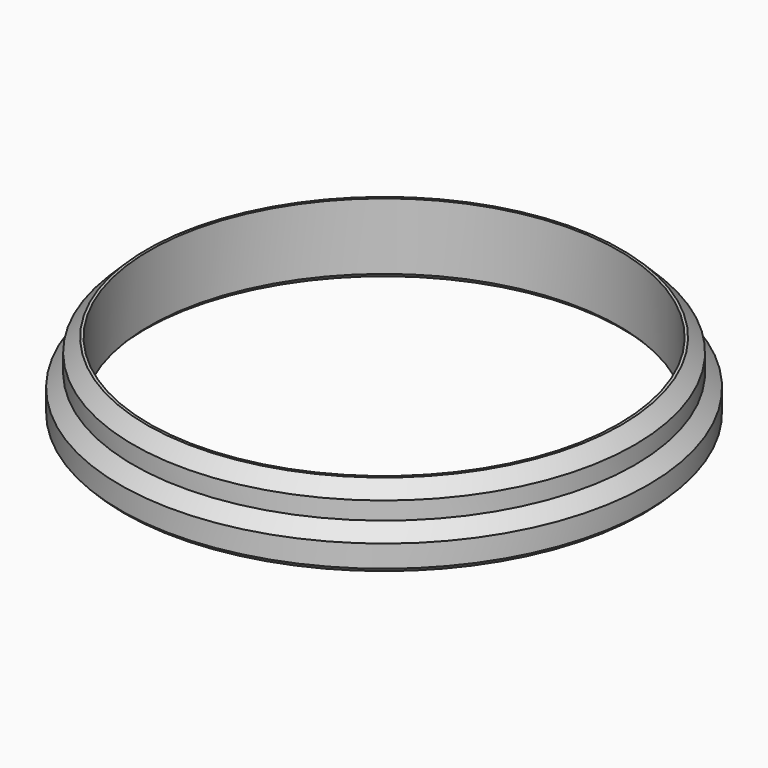
from build123d import *

# Parameters (mm, degrees)
F0_R     = 28.3
F0_R_2   = 26.5
F1_DEPTH = 8
F2_SIZE  = 1.5
F3_SIZE  = 0.5
F4_R     = 29.8
F4_R_2   = 28.3
F5_DEPTH = 4.5
F6_SIZE  = 1.49999
F7_SIZE  = 0.5


# Not quite as in the source:
# - a fillet or chamfer is up to 0.001 mm smaller than in the source, because OpenCascade refuses the exact size


with BuildPart() as f1:
    # F0 (on Top) → F1 (new body)
    with BuildSketch(Plane.XY):
        Circle(F0_R)
        Circle(F0_R_2, mode=Mode.SUBTRACT)
    extrude(amount=F1_DEPTH)

    # F2
    f2_edges = [f1.edges().sort_by_distance(p)[0] for p in [
        (-28.3, 0, 8),
    ]]
    chamfer(f2_edges, length=F2_SIZE)

    # F3
    f3_edges = [f1.edges().sort_by_distance(p)[0] for p in [
        (-26.5, 0, 0),
    ]]
    chamfer(f3_edges, length=F3_SIZE)

    # F4 (on face) → F5 (join)
    with BuildSketch(Plane(origin=(0, 0, 0), x_dir=(1, 0, 0), z_dir=(0, 0, -1))):
        Circle(F4_R)
        Circle(F4_R_2, mode=Mode.SUBTRACT)
    extrude(amount=-F5_DEPTH)

    # F6 (size 1.5 in the source; OpenCascade refuses exactly that, so slightly less here)
    f6_edges = [f1.edges().sort_by_distance(p)[0] for p in [
        (-29.8, 0, 4.5),
    ]]
    chamfer(f6_edges, length=F6_SIZE)

    # F7
    f7_edges = [f1.edges().sort_by_distance(p)[0] for p in [
        (-29.8, 0, 0),
    ]]
    chamfer(f7_edges, length=F7_SIZE)


solid = f1.part
